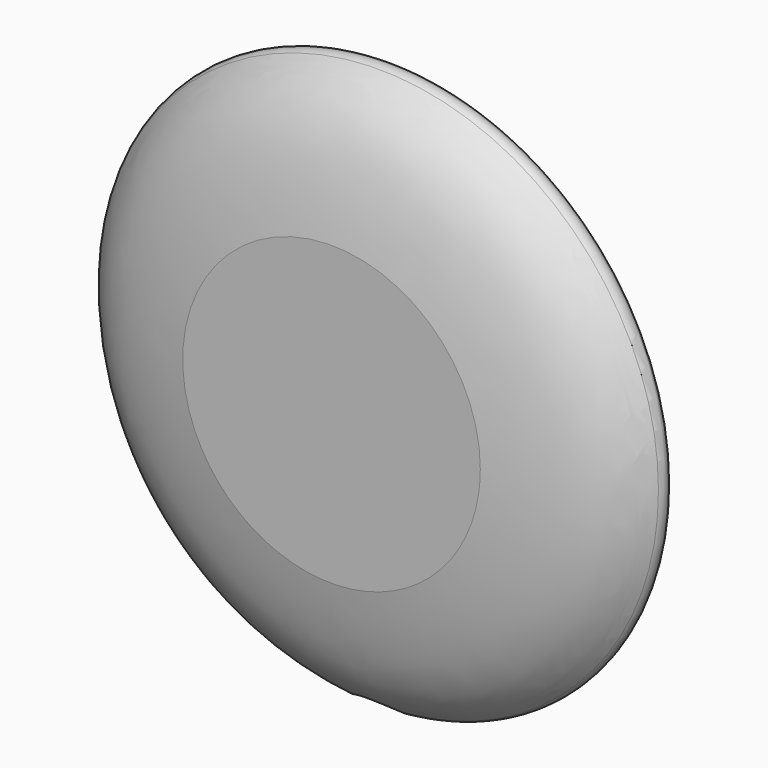
from build123d import *

# Parameters (mm, degrees)
F2_R     = 133.0483788451
F3_DEPTH = 0.8001
F5_DEPTH = 61.214


# Not quite as in the source:
# - the dataset's text gives a spline's control points without its knots; the knots are read off the source's solid


with BuildPart() as f1:
    # F0 (on Top) → F1 (revolve)
    with BuildSketch(Plane.XY):
        with BuildLine():
            Line((0, 3.175), (0, 0))
            add(Edge.make_bspline(
                [(0, 0), (1.932312764, 0), (4.4710055987, -0.0558776961), (7.6782060846, -0.1205766113), (10.1167392564, -0.1313099779), (12.2652124805, -0.0802874094), (14.1079262194, 0.0134534585), (16.0382083186, 0.1463913985), (18.5742202007, 0.3822751417), (21.7123487899, 0.7702958965), (24.8368658214, 1.257415469), (27.84236644, 1.8398038804), (30.165812066, 2.4045626027), (31.8749494748, 2.9103049867), (33.0794221608, 3.3223982148), (34.2294519284, 3.7889952757), (35.6994306745, 4.5070696881), (37.4185669263, 5.6229108448), (39.2653555392, 7.3181378878), (40.4191412795, 8.6765967542), (41.0084469063, 9.4273429275)],
                knots=[0, 0, 0, 0, 0.125, 0.1875, 0.25, 0.3125, 0.34375, 0.375, 0.4375, 0.5, 0.5625, 0.625, 0.6875, 0.71875, 0.75, 0.78125, 0.8125, 0.875, 0.9375, 1, 1, 1, 1], degree=3))
            ThreePointArc((41.0084469063, 9.4273429275), (40.7399181638, 11.6562899467), (38.5109711446, 11.3877612042))
            add(Edge.make_bspline(
                [(0, 3.175), (5.3475629671, 3.175), (12.7864845232, 2.5805427023), (31.778130468, 5.2661471984), (36.1000783741, 8.3164032549), (38.5109711446, 11.3877612042)],
                knots=[0, 0, 0, 0, 0.3387844663, 0.7216482094, 1, 1, 1, 1], degree=3))
        make_face()
    revolve(axis=Axis((0, 1.5875, 0), (0, 1, 0)))

    # F2 (on Front) → F3 (cut, symmetric)
    with BuildSketch(Plane.XZ):
        Circle(F2_R)
    extrude(amount=F3_DEPTH, both=True, mode=Mode.SUBTRACT)

    # F4 (on Top) → F5 (cut)
    with BuildSketch(Plane.XY):
        with BuildLine():
            Line((0, 7.5445573116), (0, 16.7238798654))
            ThreePointArc((0, 16.7238798654), (-4.5896612769, 12.1342185885), (0, 7.5445573116))
        make_face()
        with BuildLine():
            ThreePointArc((0, 7.5445573116), (3.2453806122, 8.8888379762), (4.5896612769, 12.1342185885))
            ThreePointArc((4.5896612769, 12.1342185885), (3.2453806122, 15.3795992007), (0, 16.7238798654))
            Line((0, 16.7238798654), (0, 7.5445573116))
        make_face()
    extrude(amount=-F5_DEPTH, mode=Mode.SUBTRACT)


solid = f1.part
